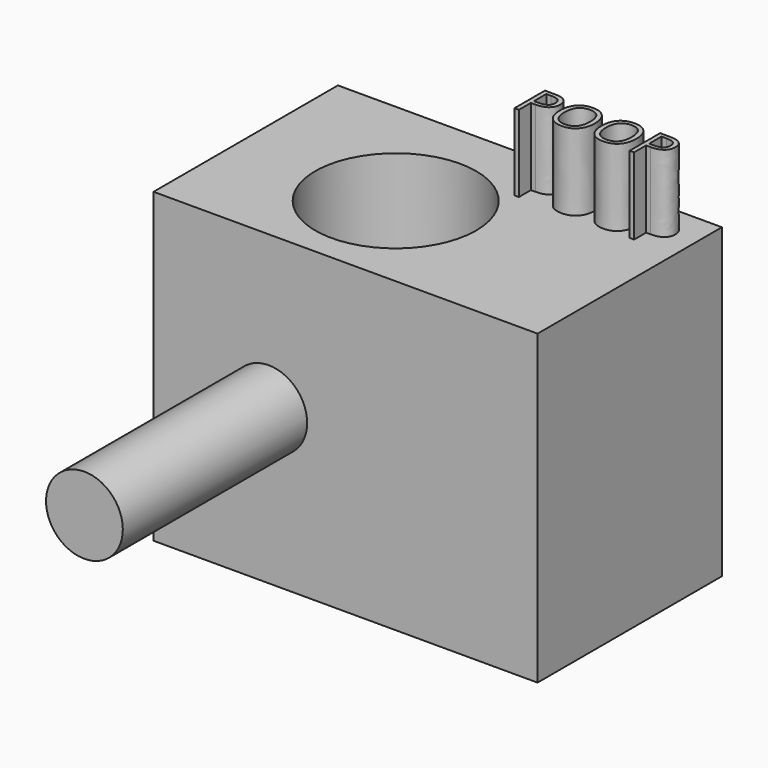
from build123d import *

# Parameters (mm, degrees)
F0_W         = 127
F0_H         = 76.2
F1_DEPTH     = 101.6
F2_R         = 12.7
F3_DEPTH     = 76.2
F4_R         = 26.6111501238
F5_DEPTH     = 101.601
F6_TEXT_SIZE = 17.6388888889
F7_DEPTH     = 25.4


# Not quite as in the source:
# - Text() gives the source's letters only with a copy of the font that has no kerning and outlines rounded to 1/6400 em; it was checked with that copy


with BuildPart() as f1:
    # F0 (on Top) → F1 (new body)
    with BuildSketch(Plane.XY):
        Rectangle(F0_W, F0_H)
    extrude(amount=F1_DEPTH)

    # F2 (on face) → F3 (join)
    with BuildSketch(Plane.XZ.offset(38.1)):
        with Locations((-25.4, 50.8)):
            Circle(F2_R)
    extrude(amount=F3_DEPTH)

    # F4 (on face) → F5 (cut, through all)
    with BuildSketch(Plane.XY.offset(101.6)):
        with Locations((-11.5051716566, -2.9919794761)):
            Circle(F4_R)
    extrude(amount=-F5_DEPTH, mode=Mode.SUBTRACT)

    # F6 (on face) → F7 (join)
    with BuildSketch(Plane.XY.offset(101.6)):
        with Locations((8.8211021081, 18.5336754337)):
            Text('POOP', F6_TEXT_SIZE, font='Open Sans', text_align=(TextAlign.LEFT, TextAlign.BOTTOM))
    extrude(amount=F7_DEPTH)


solid = f1.part
